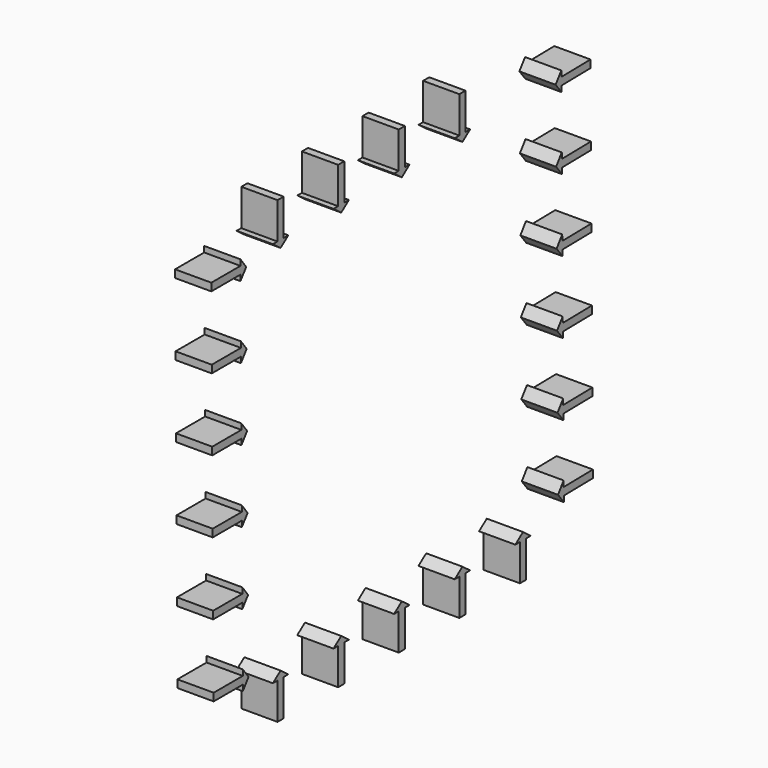
from build123d import *

# Parameters (mm, degrees)
F1_DEPTH = 1


# Not quite as in the source:
# - a feature names something its author has since deleted; it is built from what else it names


with BuildPart() as f1:
    # F0 (on Right) → F1 (new body)
    with BuildSketch(Plane.YZ):
        Polygon((-0.733841823, -10.7587281415), (0.2710369828, -10.7587281415), (0.2710369828, -10.9187281415), (0.470318177, -10.6527381415), (0.271038177, -10.3867481415), (0.271038177, -10.5467481415), (-0.733841823, -10.5467481415), align=None)
    extrude(amount=-F1_DEPTH)


with BuildPart() as f1b:
    # F0 (on Right) → F1, piece 2 (new body)
    with BuildSketch(Plane.YZ):
        Polygon((1.3094237074, -11.1468675475), (1.4694237074, -11.1468675475), (1.4694237074, -12.1517463532), (1.6814037074, -12.1517463532), (1.6814037074, -11.1468663532), (1.8414037074, -11.1468663532), (1.5754137074, -10.9475863532), align=None)
    extrude(amount=-F1_DEPTH)


with BuildPart() as f1c:
    # F0 (on Right) → F1, piece 3 (new body)
    with BuildSketch(Plane.YZ):
        Polygon((3.56, -11.1551211942), (3.56, -12.16), (3.77198, -12.16), (3.77198, -11.15512), (3.93198, -11.15512), (3.66599, -10.95584), (3.4, -11.1551211942), align=None)
    extrude(amount=-F1_DEPTH)


with BuildPart() as f1d:
    # F0 (on Right) → F1, piece 4 (new body)
    with BuildSketch(Plane.YZ):
        Polygon((5.6505762926, -11.163374841), (5.6505762926, -12.1682536468), (5.8625562926, -12.1682536468), (5.8625562926, -11.1633736468), (6.0225562926, -11.1633736468), (5.7565662926, -10.9640936468), (5.4905762926, -11.163374841), align=None)
    extrude(amount=-F1_DEPTH)


with BuildPart() as f1e:
    # F0 (on Right) → F1, piece 5 (new body)
    with BuildSketch(Plane.YZ):
        Polygon((7.7411525851, -11.1716284878), (7.7411525851, -12.1765072935), (7.9531325851, -12.1765072935), (7.9531325851, -11.1716272935), (8.1131325851, -11.1716272935), (7.8471425851, -10.9723472935), (7.5811525851, -11.1716284878), align=None)
    extrude(amount=-F1_DEPTH)


with BuildPart() as f1f:
    # F0 (on Right) → F1, piece 6 (new body)
    with BuildSketch(Plane.YZ):
        Polygon((9.8317288777, -11.1798821345), (9.8317288777, -12.1847609403), (10.0437088777, -12.1847609403), (10.0437088777, -11.1798809403), (10.2037088777, -11.1798809403), (9.9377188777, -10.9806009403), (9.6717288777, -11.1798821345), align=None)
    extrude(amount=-F1_DEPTH)


with BuildPart() as f1g:
    # F0 (on Right) → F1, piece 7 (new body)
    with BuildSketch(Plane.YZ):
        Polygon((11.3385786263, -10.2972756044), (11.1436250398, -10.5664526792), (11.3471805551, -10.8291860548), (11.3445937707, -10.6692069669), (12.3493412378, -10.6529606869), (12.3459140719, -10.4410083929), (11.3411654107, -10.4572546922), align=None)
    extrude(amount=-F1_DEPTH)


with BuildPart() as f1h:
    # F0 (on Right) → F1, piece 8 (new body)
    with BuildSketch(Plane.YZ):
        Polygon((11.3310223781, -8.8304579133), (11.3284355937, -8.6704788255), (12.3331830608, -8.6542325454), (12.3297558949, -8.4422802514), (11.3250072337, -8.4585265508), (11.3224204493, -8.2985474629), (11.1274668627, -8.5677245377), align=None)
    extrude(amount=-F1_DEPTH)


with BuildPart() as f1i:
    # F0 (on Right) → F1, piece 9 (new body)
    with BuildSketch(Plane.YZ):
        Polygon((11.3062622723, -6.2998193215), (11.1113086857, -6.5689963962), (11.3148642011, -6.8317297718), (11.3122774167, -6.671750684), (12.3170248838, -6.655504404), (12.3135977178, -6.44355211), (11.3088490566, -6.4597984093), align=None)
    extrude(amount=-F1_DEPTH)


with BuildPart() as f1j:
    # F0 (on Right) → F1, piece 10 (new body)
    with BuildSketch(Plane.YZ):
        Polygon((12.2974395408, -4.4448239685), (11.2926908796, -4.4610702678), (11.2901040952, -4.30109118), (11.0951505087, -4.5702682548), (11.298706024, -4.8330016304), (11.2961192397, -4.6730225425), (12.3008667068, -4.6567762625), align=None)
    extrude(amount=-F1_DEPTH)


with BuildPart() as f1k:
    # F0 (on Right) → F1, piece 11 (new body)
    with BuildSketch(Plane.YZ):
        Polygon((11.2739459182, -2.3023630385), (11.0789923317, -2.5715401133), (11.282547847, -2.8342734889), (11.2799610626, -2.6742944011), (12.2847085298, -2.658048121), (12.2812813638, -2.446095827), (11.2765327026, -2.4623421264), align=None)
    extrude(amount=-F1_DEPTH)


with BuildPart() as f1l:
    # F0 (on Right) → F1, piece 12 (new body)
    with BuildSketch(Plane.YZ):
        Polygon((11.2577877412, -0.3036348971), (11.0628341547, -0.5728119719), (11.26638967, -0.8355453474), (11.2638028856, -0.6755662596), (12.2685503527, -0.6593199796), (12.2651231868, -0.4473676856), (11.2603745256, -0.4636139849), align=None)
    extrude(amount=-F1_DEPTH)


with BuildPart() as f1m:
    # F0 (on Right) → F1, piece 13 (new body)
    with BuildSketch(Plane.YZ):
        Polygon((7.5811525851, -0.4566367399), (7.8471425851, -0.6559179341), (8.1131325851, -0.4566379341), (7.9531325851, -0.4566379341), (7.9531325851, 0.5482420659), (7.7411525851, 0.5482420659), (7.7411525851, -0.4566367399), align=None)
    extrude(amount=-F1_DEPTH)


with BuildPart() as f1n:
    # F0 (on Right) → F1, piece 14 (new body)
    with BuildSketch(Plane.YZ):
        Polygon((5.4905762926, -0.4648903866), (5.7565662926, -0.6641715809), (6.0225562926, -0.4648915809), (5.8625562926, -0.4648915809), (5.8625562926, 0.5399884191), (5.6505762926, 0.5399884191), (5.6505762926, -0.4648903866), align=None)
    extrude(amount=-F1_DEPTH)


with BuildPart() as f1o:
    # F0 (on Right) → F1, piece 15 (new body)
    with BuildSketch(Plane.YZ):
        Polygon((3.77198, 0.5317347724), (3.56, 0.5317347724), (3.56, -0.4731440334), (3.4, -0.4731440334), (3.66599, -0.6724252276), (3.93198, -0.4731452276), (3.77198, -0.4731452276), align=None)
    extrude(amount=-F1_DEPTH)


with BuildPart() as f1p:
    # F0 (on Right) → F1, piece 16 (new body)
    with BuildSketch(Plane.YZ):
        Polygon((1.4694237074, 0.5234811256), (1.4694237074, -0.4813976802), (1.3094237074, -0.4813976802), (1.5754137074, -0.6806788744), (1.8414037074, -0.4813988744), (1.6814037074, -0.4813988744), (1.6814037074, 0.5234811256), align=None)
    extrude(amount=-F1_DEPTH)


with BuildPart() as f1q:
    # F0 (on Right) → F1, piece 17 (new body)
    with BuildSketch(Plane.YZ):
        Polygon((0.1902472919, -0.5531074341), (-0.8146327081, -0.5531074341), (-0.8146327081, -0.7650874341), (0.1902460977, -0.7650874341), (0.1902460977, -0.9250874341), (0.3895272919, -0.6590974341), (0.1902472919, -0.3931074341), align=None)
    extrude(amount=-F1_DEPTH)


with BuildPart() as f1r:
    # F0 (on Right) → F1, piece 18 (new body)
    with BuildSketch(Plane.YZ):
        Polygon((0.2064054689, -2.5518355756), (-0.7984745311, -2.5518355756), (-0.7984745311, -2.7638155756), (0.2064042747, -2.7638155756), (0.2064042747, -2.9238155756), (0.4056854689, -2.6578255756), (0.2064054689, -2.3918355756), align=None)
    extrude(amount=-F1_DEPTH)


with BuildPart() as f1s:
    # F0 (on Right) → F1, piece 19 (new body)
    with BuildSketch(Plane.YZ):
        Polygon((0.222563646, -4.5505637171), (-0.782316354, -4.5505637171), (-0.782316354, -4.7625437171), (0.2225624517, -4.7625437171), (0.2225624517, -4.9225437171), (0.421843646, -4.6565537171), (0.222563646, -4.3905637171), align=None)
    extrude(amount=-F1_DEPTH)


with BuildPart() as f1t:
    # F0 (on Right) → F1, piece 20 (new body)
    with BuildSketch(Plane.YZ):
        Polygon((0.238721823, -6.5492918585), (-0.766158177, -6.5492918585), (-0.766158177, -6.7612718585), (0.2387206288, -6.7612718585), (0.2387206288, -6.9212718585), (0.438001823, -6.6552818585), (0.238721823, -6.3892918585), align=None)
    extrude(amount=-F1_DEPTH)


with BuildPart() as f1u:
    # F0 (on Right) → F1, piece 21 (new body)
    with BuildSketch(Plane.YZ):
        Polygon((0.25488, -8.54802), (-0.75, -8.54802), (-0.75, -8.76), (0.2548788058, -8.76), (0.2548788058, -8.92), (0.45416, -8.65401), (0.25488, -8.38802), align=None)
    extrude(amount=-F1_DEPTH)


solid = Compound([f1.part, f1b.part, f1c.part, f1d.part, f1e.part, f1f.part, f1g.part, f1h.part, f1i.part, f1j.part, f1k.part, f1l.part, f1m.part, f1n.part, f1o.part, f1p.part, f1q.part, f1r.part, f1s.part, f1t.part, f1u.part])
